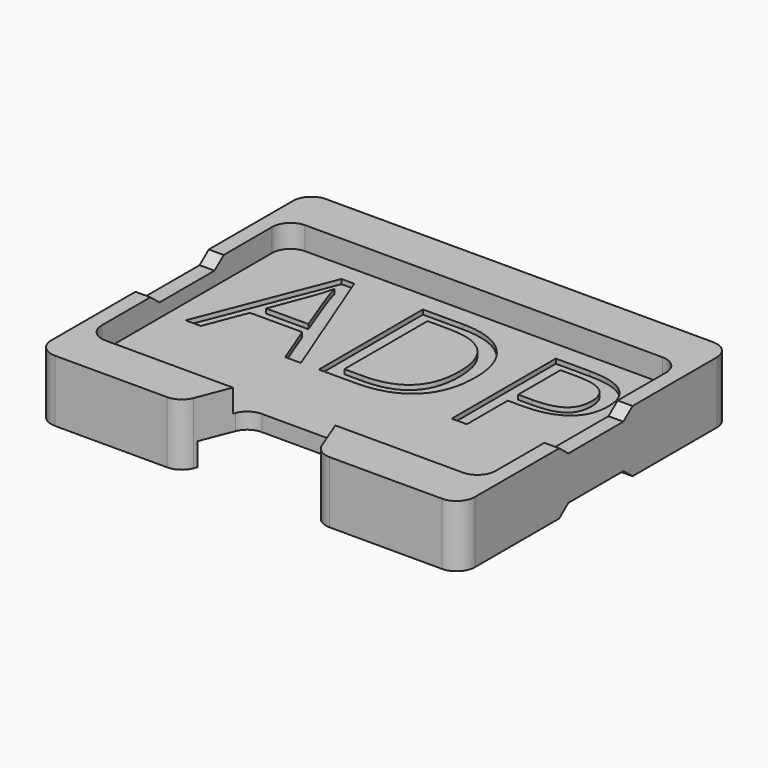
from build123d import *

# Parameters (mm, degrees)
F2_DEPTH      = 8.5
F2_DEPTH_BACK = 5
F3_DEPTH      = 5
F5_START      = -3.5
F5_DEPTH      = 5
F7_DEPTH      = 5
F7_DEPTH_BACK = 8.5
F8_R          = 4
F9_TEXT_SIZE  = 39.7944089725
F10_DEPTH     = 1
F12_DEPTH     = 92.501


# Not quite as in the source:
# - Text() gives the source's letters only with a copy of the font that has no kerning and outlines rounded to 1/6400 em; it was checked with that copy


with BuildPart() as f2:
    # F1 (on Top) → F2 (new body, two sides)
    with BuildSketch(Plane.XY) as f2_sk:
        with BuildLine():
            ThreePointArc((-3.25, -5.75), (-2.0784271247, -8.5784271247), (0.75, -9.75))
            Line((0.75, -9.75), (85.25, -9.75))
            ThreePointArc((85.25, -9.75), (88.0784271247, -8.5784271247), (89.25, -5.75))
            Line((89.25, -5.75), (89.25, 60.25))
            ThreePointArc((89.25, 60.25), (88.0784271247, 63.0784271247), (85.25, 64.25))
            Line((85.25, 64.25), (0.75, 64.25))
            ThreePointArc((0.75, 64.25), (-2.0784271247, 63.0784271247), (-3.25, 60.25))
            Line((-3.25, 60.25), (-3.25, -5.75))
        make_face()
    extrude(amount=-F2_DEPTH)
    extrude(f2_sk.sketch, amount=F2_DEPTH_BACK)

    # F0 (on Top) → F3 (cut)
    with BuildSketch(Plane.XY):
        with BuildLine():
            ThreePointArc((0, 4), (1.1715728753, 1.1715728753), (4, 0))
            Line((4, 0), (82, 0))
            ThreePointArc((82, 0), (84.8284271247, 1.1715728753), (86, 4))
            Line((86, 4), (86, 50.5))
            ThreePointArc((86, 50.5), (84.8284271247, 53.3284271247), (82, 54.5))
            Line((82, 54.5), (4, 54.5))
            ThreePointArc((4, 54.5), (1.1715728753, 53.3284271247), (0, 50.5))
            Line((0, 50.5), (0, 4))
        make_face()
    extrude(amount=F3_DEPTH, mode=Mode.SUBTRACT)

    # F4 (on Top) → F5 (cut)
    with BuildSketch(Plane.XY.offset(F5_START)):
        with BuildLine():
            ThreePointArc((0, -2.5), (1.1715728753, -5.3284271247), (4, -6.5))
            Line((4, -6.5), (81.9533548355, -6.5))
            ThreePointArc((81.9533548355, -6.5), (84.7817819603, -5.3284271247), (85.9533548355, -2.5))
            Line((85.9533548355, -2.5), (85.9533548355, 56.7386844754))
            ThreePointArc((85.9533548355, 56.7386844754), (84.7817819603, 59.5671116002), (81.9533548355, 60.7386844754))
            Line((81.9533548355, 60.7386844754), (4, 60.7386844754))
            ThreePointArc((4, 60.7386844754), (1.1715728753, 59.5671116002), (0, 56.7386844754))
            Line((0, 56.7386844754), (0, -2.5))
        make_face()
    extrude(amount=-F5_DEPTH, mode=Mode.SUBTRACT)

    # F6 (on Top) → F7 (cut, two sides)
    with BuildSketch(Plane.XY) as f7_sk:
        with BuildLine():
            Line((32.0040588687, 0.4603501153), (28, -9.75))
            Line((28, -9.75), (43, -9.75))
            Line((43, -9.75), (58, -9.75))
            Line((58, -9.75), (53.9959411313, 0.4603501153))
            ThreePointArc((53.9959411313, 0.4603501153), (52.5257785273, 2.3046482764), (50.2720483373, 3))
            Line((50.2720483373, 3), (43, 3))
            Line((43, 3), (35.7279516627, 3))
            ThreePointArc((35.7279516627, 3), (33.4742214727, 2.3046482764), (32.0040588687, 0.4603501153))
        make_face()
    extrude(amount=F7_DEPTH, mode=Mode.SUBTRACT)
    extrude(f7_sk.sketch, amount=-F7_DEPTH_BACK, mode=Mode.SUBTRACT)

    # F8
    f8_edges = [f2.edges().sort_by_distance(p)[0] for p in [
        (58, -9.75, -1.75),
        (28, -9.75, -1.75),
    ]]
    fillet(f8_edges, radius=F8_R)

    # F9 (on face) → F10 (cut)
    with BuildSketch(Plane.XY):
        with Locations((4, 21.8480255398)):
            Text('ADP', F9_TEXT_SIZE, font='Open Sans', text_align=(TextAlign.LEFT, TextAlign.BOTTOM))
    extrude(amount=-F10_DEPTH, mode=Mode.SUBTRACT)

    # F11 (on face) → F12 (cut, through all)
    with BuildSketch(Plane(origin=(-3.25, 0, 0), x_dir=(0, -1, 0), z_dir=(-1, 0, 0))):
        Polygon((-19.75, 3), (-17.25, 5), (-27.25, 5), (-37.25, 5), (-34.75, 3), (-27.25, 3), align=None)
        Polygon((-27.25, -8.5), (-17.25, -8.5), (-19.75, -6.5), (-27.25, -6.5), (-34.75, -6.5), (-37.25, -8.5), align=None)
    extrude(amount=-F12_DEPTH, mode=Mode.SUBTRACT)


solid = f2.part
